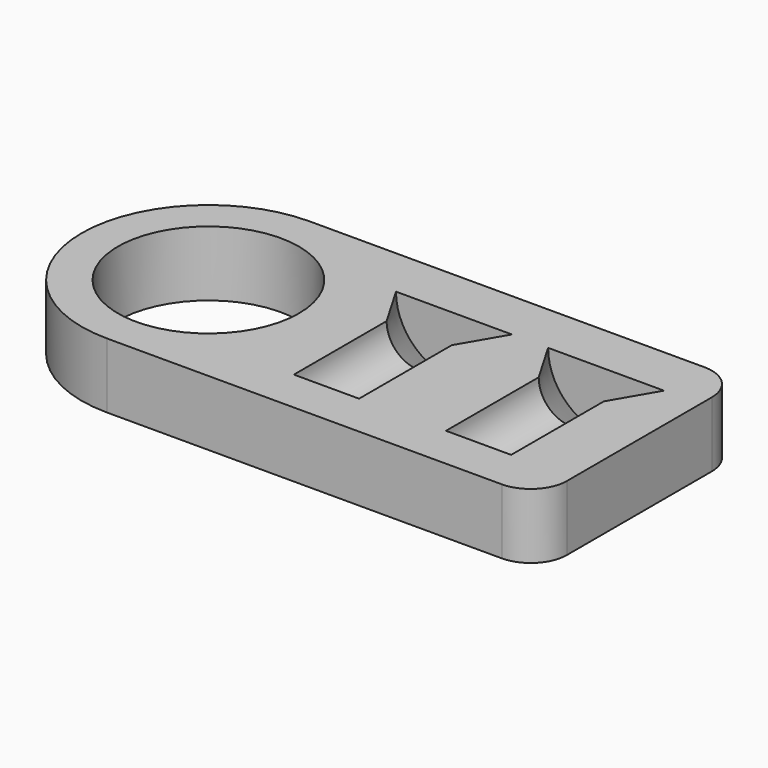
from build123d import *

# Parameters (mm, degrees)
F0_R         = 12.5
F1_DEPTH     = 9
F5_TEXT_SIZE = 5.5555555556
F6_DEPTH     = 1


# Not quite as in the source:
# - Text() gives the source's letters only with a copy of the font that has no kerning and outlines rounded to 1/6400 em; it was checked with that copy


with BuildPart() as f1:
    # F0 (on Top) → F1 (new body)
    with BuildSketch(Plane.XY):
        with BuildLine():
            ThreePointArc((0, 17.5), (5.1256313292, 5.1256313292), (17.5, 0))
            Line((17.5, 0), (72, 0))
            ThreePointArc((72, 0), (75.5355339059, 1.4644660941), (77, 5))
            Line((77, 5), (77, 30))
            ThreePointArc((77, 30), (75.5355339059, 33.5355339059), (72, 35))
            Line((72, 35), (17.5, 35))
            ThreePointArc((17.5, 35), (5.1256313292, 29.8743686708), (0, 17.5))
        make_face()
        with Locations((17.5, 17.5)):
            Circle(F0_R, mode=Mode.SUBTRACT)
    extrude(amount=F1_DEPTH)

    # F2 (on face) → F3 (revolve, cut)
    with BuildSketch(Plane.XY.offset(9)):
        Polygon((43, 28), (43, 6), (47.5, 6), (47.5, 22), (51, 28), align=None)
    revolve(axis=Axis((43, 17, 9), (0, 1, 0)), mode=Mode.SUBTRACT)

    # F2 (on face) → F4 (revolve, cut)
    with BuildSketch(Plane.XY.offset(9)):
        Polygon((64, 28), (64, 6), (68.5, 6), (68.5, 22), (72, 28), align=None)
    revolve(axis=Axis((64, 17, 9), (0, 1, 0)), mode=Mode.SUBTRACT)

    # F5 (on face) → F6 (cut)
    with BuildSketch(Plane(origin=(0, 0, 0), x_dir=(1, 0, 0), z_dir=(0, 0, -1))):
        with Locations((30, -9)):
            Text('824, 825', F5_TEXT_SIZE, font='Open Sans', text_align=(TextAlign.LEFT, TextAlign.BOTTOM))
    extrude(amount=-F6_DEPTH, mode=Mode.SUBTRACT)


solid = f1.part
